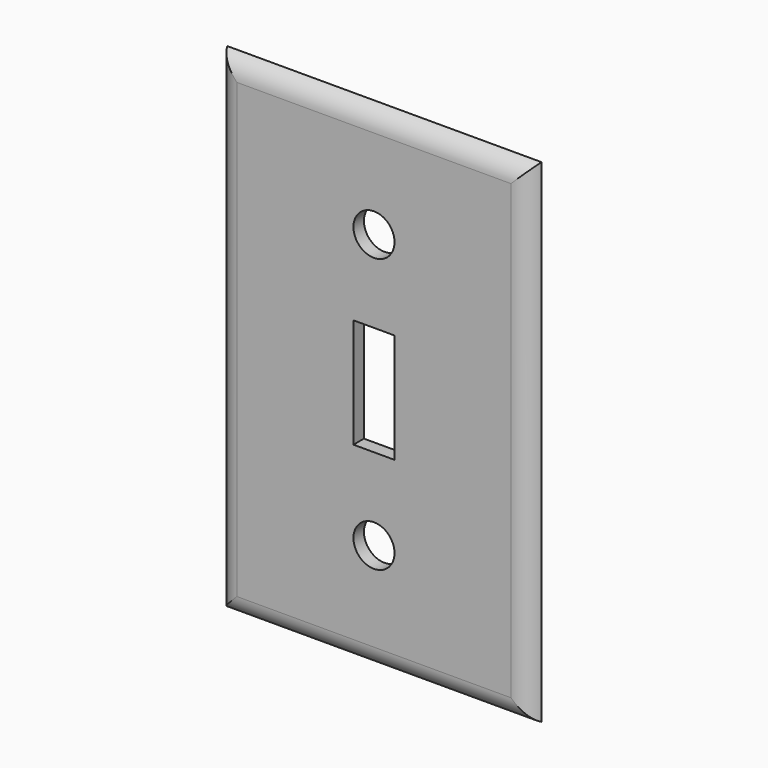
from build123d import *

# Parameters (mm, degrees)
F0_W        = 72.898
F0_H        = 114.3
F0_R        = 4.7625
F0_W_2      = 9.525
F0_H_2      = 25.4
F1_DEPTH    = 3.048
F2_T1_DEPTH = 96.1774845304
F2_T3_DEPTH = 137.5794845304


# Not quite as in the source:
# - a fillet or chamfer that OpenCascade refuses, or shapes differently, is made with other operations: its cross-section is extruded or revolved along the edge and cut away or added


with BuildPart() as f1:
    # F0 (on Front) → F1 (new body)
    with BuildSketch(Plane.XZ):
        Rectangle(F0_W, F0_H)
        with Locations((0, -31.75)):
            Circle(F0_R, mode=Mode.SUBTRACT)
        Rectangle(F0_W_2, F0_H_2, mode=Mode.SUBTRACT)
        with Locations((0, 31.75)):
            Circle(F0_R, mode=Mode.SUBTRACT)
    extrude(amount=F1_DEPTH)

    # F2: fillet of radius 5.08 on 4 edges, made by hand

    # F2_s2 → F2_t1 (cut)
    with BuildSketch(Plane.YZ.offset(-48.0887422652)):
        with BuildLine():
            ThreePointArc((0, 57.15), (-2.2182329348, 55.2765336861), (-3.048, 52.4941030939))
            Line((-3.048, 52.4941030939), (-3.048, 57.15))
            Line((-3.048, 57.15), (0, 57.15))
        make_face()
        with BuildLine():
            ThreePointArc((0, -57.15), (-2.2182329348, -55.2765336861), (-3.048, -52.4941030939))
            Line((-3.048, -52.4941030939), (-3.048, -57.15))
            Line((-3.048, -57.15), (0, -57.15))
        make_face()
    extrude(amount=F2_T1_DEPTH, mode=Mode.SUBTRACT)

    # F2_s4 → F2_t3 (cut)
    with BuildSketch(Plane.XY.offset(-68.7897422652)):
        with BuildLine():
            ThreePointArc((36.449, 0), (34.5755336861, -2.2182329348), (31.7931030939, -3.048))
            Line((31.7931030939, -3.048), (36.449, -3.048))
            Line((36.449, -3.048), (36.449, 0))
        make_face()
        with BuildLine():
            ThreePointArc((-36.449, 0), (-34.5755336861, -2.2182329348), (-31.7931030939, -3.048))
            Line((-31.7931030939, -3.048), (-36.449, -3.048))
            Line((-36.449, -3.048), (-36.449, 0))
        make_face()
    extrude(amount=F2_T3_DEPTH, mode=Mode.SUBTRACT)


solid = f1.part
